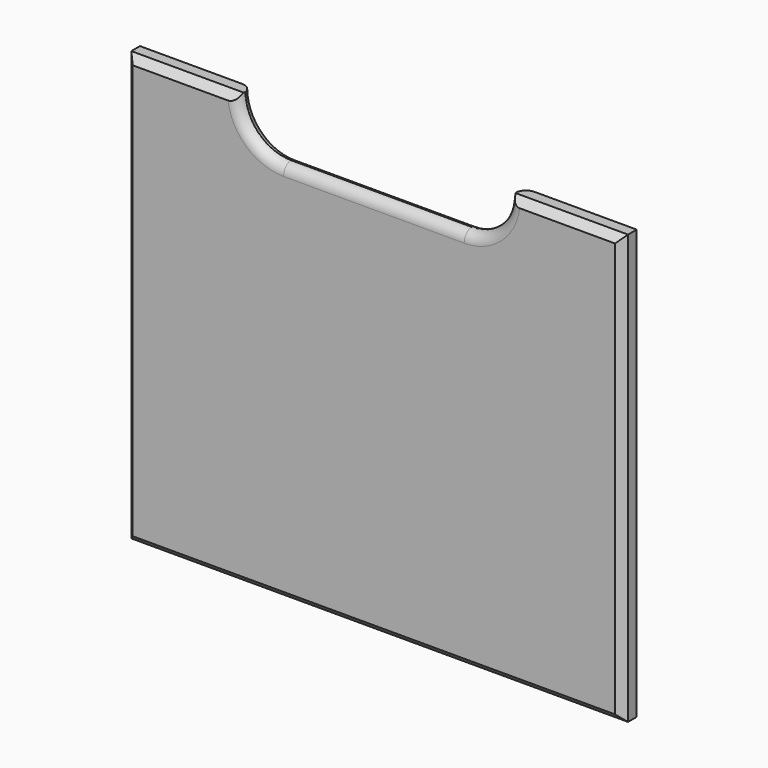
from build123d import *

# Parameters (mm, degrees)
F1_DEPTH     = 12.7
F2_T1_DEPTH  = 127
F2_T4_ANGLE  = 124.391277417
F2_T6_ANGLE  = 124.391277417
F2_T8_ANGLE  = 124.391277417
F2_T10_ANGLE = 124.391277417
F3_T1_DEPTH  = 97.8832991577
F3_T3_DEPTH  = 327.7532991577
F3_T5_DEPTH  = 375.3782991577
F3_T7_DEPTH  = 97.8832991577


# Not quite as in the source:
# - a fillet or chamfer that OpenCascade refuses, or shapes differently, is made with other operations: its cross-section is extruded or revolved along the edge and cut away or added


with BuildPart() as f1:
    # F0 (on Front) → F1 (new body)
    with BuildSketch(Plane.XZ):
        with BuildLine():
            Line((-95.25, 80.8194016659), (-174.625, 80.8194016659))
            Line((-174.625, 80.8194016659), (-174.625, -220.8055983341))
            Line((-174.625, -220.8055983341), (174.625, -220.8055983341))
            Line((174.625, -220.8055983341), (174.625, 80.8194016659))
            Line((174.625, 80.8194016659), (95.25, 80.8194016659))
            ThreePointArc((95.25, 80.8194016659), (85.9506403027, 58.3687613632), (63.5, 49.0694016659))
            Line((63.5, 49.0694016659), (-63.5, 49.0694016659))
            ThreePointArc((-63.5, 49.0694016659), (-85.9506403027, 58.3687613632), (-95.25, 80.8194016659))
        make_face()
    extrude(amount=F1_DEPTH)

    # F2: fillet of radius 7.62 on 6 edges, made by hand

    # F2_s2 → F2_t1 (cut)
    with BuildSketch(Plane.YZ.offset(-63.5)):
        with BuildLine():
            ThreePointArc((-5.08, 49.0694016659), (-10.4681536726, 46.8375553385), (-12.7, 41.4494016659))
            Line((-12.7, 41.4494016659), (-12.7, 49.0694016659))
            Line((-12.7, 49.0694016659), (-5.08, 49.0694016659))
        make_face()
        with BuildLine():
            ThreePointArc((-7.62, 49.0694016659), (-2.2318463274, 46.8375553385), (0, 41.4494016659))
            Line((0, 41.4494016659), (0, 49.0694016659))
            Line((0, 49.0694016659), (-7.62, 49.0694016659))
        make_face()
    extrude(amount=F2_T1_DEPTH, mode=Mode.SUBTRACT)

    # F2_s3 → F2_t4 (revolve, cut)
    with BuildSketch(Plane(origin=(-17.4110672308, 0, 25.4365284857), x_dir=(0, 1, 0), z_dir=(-0.5648413834, 0, 0.825199498))):
        with BuildLine():
            ThreePointArc((-7.62, -129.8003107701), (-2.2318463274, -132.0321570975), (0, -137.4203107701))
            Line((0, -137.4203107701), (0, -129.8003107701))
            Line((0, -129.8003107701), (-7.62, -129.8003107701))
        make_face()
    revolve(axis=Axis((63.5, 0, 80.8194016659), (0, 1, 0)), revolution_arc=F2_T4_ANGLE, mode=Mode.SUBTRACT)

    # F2_s5 → F2_t6 (revolve, cut)
    with BuildSketch(Plane(origin=(-17.4110672308, 0, 25.4365284857), x_dir=(0, 1, 0), z_dir=(-0.5648413834, 0, 0.825199498))):
        with BuildLine():
            ThreePointArc((-5.08, -129.8003107701), (-10.4681536726, -132.0321570975), (-12.7, -137.4203107701))
            Line((-12.7, -137.4203107701), (-12.7, -129.8003107701))
            Line((-12.7, -129.8003107701), (-5.08, -129.8003107701))
        make_face()
    revolve(axis=Axis((63.5, -12.7, 80.8194016659), (0, 1, 0)), revolution_arc=F2_T6_ANGLE, mode=Mode.SUBTRACT)

    # F2_s7 → F2_t8 (revolve, cut)
    with BuildSketch(Plane.YZ.offset(-63.5)):
        with BuildLine():
            ThreePointArc((-7.62, 49.0694016659), (-2.2318463274, 46.8375553385), (0, 41.4494016659))
            Line((0, 41.4494016659), (0, 49.0694016659))
            Line((0, 49.0694016659), (-7.62, 49.0694016659))
        make_face()
    revolve(axis=Axis((-63.5, 0, 80.8194016659), (0, 1, 0)), revolution_arc=F2_T8_ANGLE, mode=Mode.SUBTRACT)

    # F2_s9 → F2_t10 (revolve, cut)
    with BuildSketch(Plane.YZ.offset(-63.5)):
        with BuildLine():
            ThreePointArc((-5.08, 49.0694016659), (-10.4681536726, 46.8375553385), (-12.7, 41.4494016659))
            Line((-12.7, 41.4494016659), (-12.7, 49.0694016659))
            Line((-12.7, 49.0694016659), (-5.08, 49.0694016659))
        make_face()
    revolve(axis=Axis((-63.5, -12.7, 80.8194016659), (0, 1, 0)), revolution_arc=F2_T10_ANGLE, mode=Mode.SUBTRACT)

    # F3: chamfer of 5.08 on 5 edges, made by hand

    # F3_s2 → F3_t1 (cut)
    with BuildSketch(Plane.YZ.offset(-187.6891495789)):
        Polygon((-7.62, 80.8194016659), (-12.7, 75.7394016659), (-12.7, 80.8194016659), align=None)
    extrude(amount=F3_T1_DEPTH, mode=Mode.SUBTRACT)

    # F3_s4 → F3_t3 (cut)
    with BuildSketch(Plane.XY.offset(-233.869747913)):
        Polygon((-174.625, -7.62), (-169.545, -12.7), (-174.625, -12.7), align=None)
        Polygon((169.545, -12.7), (174.625, -7.62), (174.625, -12.7), align=None)
    extrude(amount=F3_T3_DEPTH, mode=Mode.SUBTRACT)

    # F3_s6 → F3_t5 (cut)
    with BuildSketch(Plane.YZ.offset(-187.6891495789)):
        Polygon((-12.7, -215.7255983341), (-7.62, -220.8055983341), (-12.7, -220.8055983341), align=None)
    extrude(amount=F3_T5_DEPTH, mode=Mode.SUBTRACT)

    # F3_s8 → F3_t7 (cut)
    with BuildSketch(Plane.YZ.offset(89.8058504211)):
        Polygon((-12.7, 75.7394016659), (-7.62, 80.8194016659), (-12.7, 80.8194016659), align=None)
    extrude(amount=F3_T7_DEPTH, mode=Mode.SUBTRACT)


solid = f1.part
